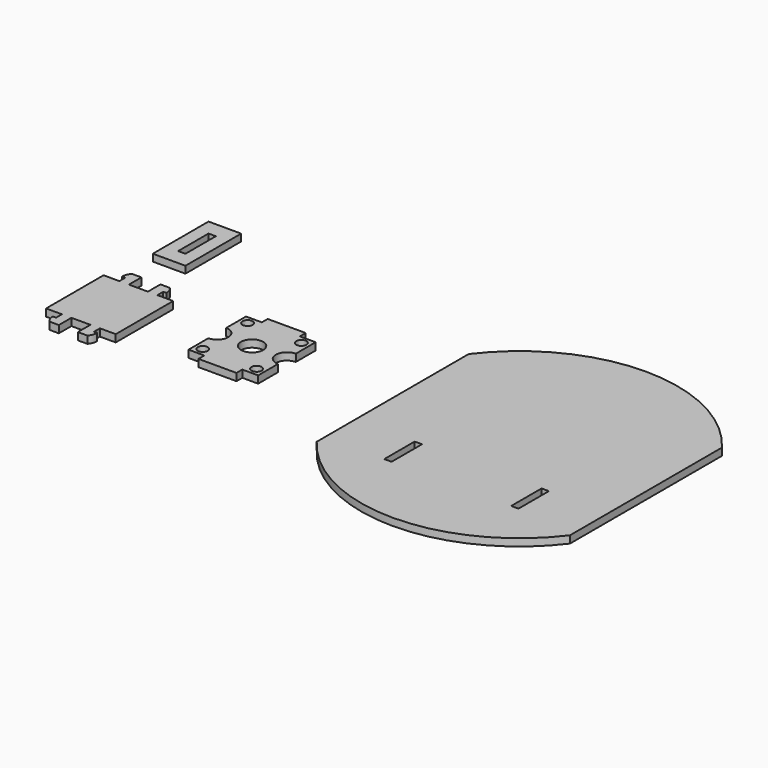
from build123d import *

# Parameters (mm, degrees)
F0_W      = 22
F0_H      = 22.7
F1_DEPTH  = 2.3114
F3_D      = 3.2
F4_W      = 12
F4_H      = 2.3114
F5_DEPTH  = 2.3114
F8_D      = 7
F10_DEPTH = 2.3114
F11_W     = 2.3114
F11_H     = 12
F12_DEPTH = 2.3124
F13_W     = 5
F13_H     = 11.35
F13_W_2   = 3
F14_DEPTH = 2.3114
F15_W     = 10.311
F15_H     = 22
F15_W_2   = 2.3114
F15_H_2   = 12
F16_DEPTH = 2.211


# Not quite as in the source:
# - a feature names something its author has since deleted; it is built from what else it names


with BuildPart() as f1:
    # F0 (on Top) → F1 (new body)
    with BuildSketch(Plane.XY):
        Rectangle(F0_W, F0_H)
    extrude(amount=F1_DEPTH)

    # F3 (through all)
    with Locations(Plane.XY.offset(2.3114)):
        with Locations((-8.5, 8.85), (8.5, 8.85), (8.5, -8.85), (-8.5, -8.85)):
            Hole(F3_D / 2)


with BuildPart() as f5:
    # F4 (on face) → F5 (new body)
    with BuildSketch(Plane.XY.offset(2.3114)):
        with Locations((0, 12.5057)):
            Rectangle(F4_W, F4_H)
    extrude(amount=-F5_DEPTH)


with BuildPart() as f5b:
    # F4 (on face) → F5, piece 2 (new body)
    with BuildSketch(Plane.XY.offset(2.3114)):
        with Locations((0, -12.5057)):
            Rectangle(F4_W, F4_H)
    extrude(amount=-F5_DEPTH)


with BuildPart() as f1_1:
    add(f1.part)

    # F6: union F5, F5b
    add(f5.part)
    add(f5b.part)

    # F8 (through all)
    with Locations(Plane.XY.offset(2.3114)):
        with Locations((-11, 0), (11, 0), (0, 0)):
            Hole(F8_D / 2)


with BuildPart() as f10:
    # F9 (on Top) → F10 (new body)
    with BuildSketch(Plane.XY):
        with BuildLine():
            Line((124.4197436075, -30), (124.4197436075, 30))
            ThreePointArc((124.4197436075, 30), (106.7804233825, 44.72135955), (84.4197436075, 50))
            ThreePointArc((84.4197436075, 50), (62.0590638325, 44.72135955), (44.4197436075, 30))
            Line((44.4197436075, 30), (44.4197436075, -30))
            ThreePointArc((44.4197436075, -30), (62.0590638325, -44.72135955), (84.4197436075, -50))
            ThreePointArc((84.4197436075, -50), (106.7804233825, -44.72135955), (124.4197436075, -30))
        make_face()
    extrude(amount=F10_DEPTH)

    # F11 (on face) → F12 (cut, through all)
    with BuildSketch(Plane.XY.offset(2.3114)):
        with Locations((64.3754436075, -20.8296453593)):
            Rectangle(F11_W, F11_H)
        with Locations((104.4640436075, -20.8296453593)):
            Rectangle(F11_W, F11_H)
    extrude(amount=-F12_DEPTH, mode=Mode.SUBTRACT)


with BuildPart() as f14:
    # F13 (on Top) → F14 (new body)
    with BuildSketch(Plane.XY):
        with Locations((-49.6969209611, 0.9244190347)):
            Rectangle(F13_W, F13_H)
        with Locations((-45.6969209611, 0.9244190347)):
            Rectangle(F13_W_2, F13_H)
        with Locations((-39.6969209611, 0.9244190347)):
            Rectangle(F13_W_2, F13_H)
        with Locations((-39.6969209611, -10.4255809653)):
            Rectangle(F13_W_2, F13_H)
        with Locations((-49.6969209611, -10.4255809653)):
            Rectangle(F13_W, F13_H)
        with Locations((-32.6969209611, -10.4255809653)):
            Rectangle(F13_W, F13_H)
        with Locations((-32.6969209611, 0.9244190347)):
            Rectangle(F13_W, F13_H)
        with BuildLine():
            Line((-35.1969209611, -16.1005809653), (-38.1969209611, -16.1005809653))
            Line((-38.1969209611, -16.1005809653), (-38.1969209611, -18.4119809653))
            Line((-38.1969209611, -18.4119809653), (-38.1969209611, -21.0577322764))
            Line((-38.1969209611, -21.0577322764), (-35.1969209611, -21.0577322764))
            ThreePointArc((-35.1969209611, -21.0577322764), (-34.4552635744, -19.8261945277), (-34.1969209611, -18.4119809653))
            Line((-34.1969209611, -18.4119809653), (-35.1969209611, -18.4119809653))
            Line((-35.1969209611, -18.4119809653), (-35.1969209611, -16.1005809653))
        make_face()
        with Locations((-45.6969209611, -10.4255809653)):
            Rectangle(F13_W_2, F13_H)
        with Locations((-36.6969209611, 0.9244190347)):
            Rectangle(F13_W_2, F13_H)
        with Locations((-42.6969209611, 0.9244190347)):
            Rectangle(F13_W_2, F13_H)
        with Locations((-42.6969209611, -10.4255809653)):
            Rectangle(F13_W_2, F13_H)
        with Locations((-36.6969209611, -10.4255809653)):
            Rectangle(F13_W_2, F13_H)
        with BuildLine():
            Line((-47.1969209611, 8.9108190347), (-47.1969209611, 6.5994190347))
            Line((-47.1969209611, 6.5994190347), (-44.1969209611, 6.5994190347))
            Line((-44.1969209611, 6.5994190347), (-44.1969209611, 8.9108190347))
            Line((-44.1969209611, 8.9108190347), (-44.1969209611, 11.5565703458))
            Line((-44.1969209611, 11.5565703458), (-47.1969209611, 11.5565703458))
            ThreePointArc((-47.1969209611, 11.5565703458), (-47.9385783479, 10.3250325971), (-48.1969209611, 8.9108190347))
            Line((-48.1969209611, 8.9108190347), (-47.1969209611, 8.9108190347))
        make_face()
        with BuildLine():
            Line((-38.1969209611, 8.9108190347), (-38.1969209611, 6.5994190347))
            Line((-38.1969209611, 6.5994190347), (-35.1969209611, 6.5994190347))
            Line((-35.1969209611, 6.5994190347), (-35.1969209611, 8.9108190347))
            Line((-35.1969209611, 8.9108190347), (-34.1969209611, 8.9108190347))
            ThreePointArc((-34.1969209611, 8.9108190347), (-34.4552635744, 10.3250325971), (-35.1969209611, 11.5565703458))
            Line((-35.1969209611, 11.5565703458), (-38.1969209611, 11.5565703458))
            Line((-38.1969209611, 11.5565703458), (-38.1969209611, 8.9108190347))
        make_face()
        with BuildLine():
            Line((-44.1969209611, -16.1005809653), (-47.1969209611, -16.1005809653))
            Line((-47.1969209611, -16.1005809653), (-47.1969209611, -18.4119809653))
            Line((-47.1969209611, -18.4119809653), (-48.1969209611, -18.4119809653))
            ThreePointArc((-48.1969209611, -18.4119809653), (-47.9385783479, -19.8261945277), (-47.1969209611, -21.0577322764))
            Line((-47.1969209611, -21.0577322764), (-44.1969209611, -21.0577322764))
            Line((-44.1969209611, -21.0577322764), (-44.1969209611, -18.4119809653))
            Line((-44.1969209611, -18.4119809653), (-44.1969209611, -16.1005809653))
        make_face()
    extrude(amount=F14_DEPTH)


with BuildPart() as f16:
    # F15 (on Top) → F16 (new body)
    with BuildSketch(Plane.XY):
        with Locations((-44.8737465275, 34.3274882433)):
            Rectangle(F15_W, F15_H)
        with Locations((-44.8739465275, 34.3274882433)):
            Rectangle(F15_W_2, F15_H_2, mode=Mode.SUBTRACT)
    extrude(amount=F16_DEPTH)


solid = Compound([f1_1.part, f10.part, f14.part, f16.part])
